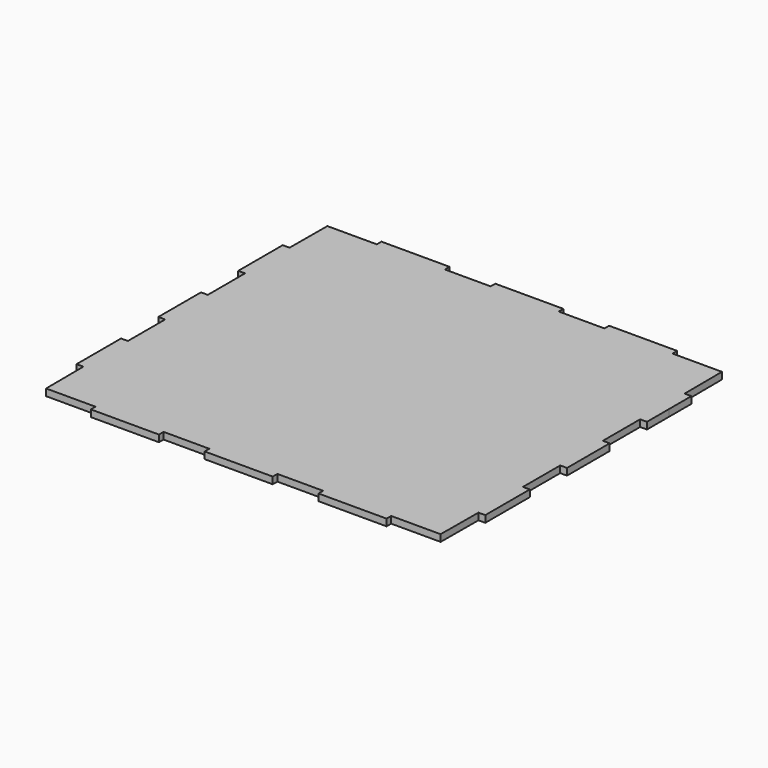
from build123d import *

# Parameters (mm, degrees)
F1_DEPTH = 3


# Not quite as in the source:
# - ends of sketch curves that miss each other by under 0.0002 mm in the source are joined


with BuildPart() as f1:
    # F0 (on Top) → F1 (new body)
    with BuildSketch(Plane.XY):
        Polygon((90.0000515607, 56.7499991818), (87.0000515607, 56.7499991818), (86.8757655059, 77.438837362), (65.1257655059, 77.4387894966), (65.1257655059, 80), (35.1257655059, 80), (35.1257655059, 77.4387894966), (15, 77.4393804423), (15, 80), (-15, 80), (-15, 77.4393804423), (-35.1257655059, 77.4387894966), (-35.1257655059, 80), (-65.1257655059, 80), (-65.1257655059, 77.4387894966), (-86.8757655059, 77.438837362), (-87.0000515607, 56.7499991818), (-90.0000515607, 56.7499991818), (-90.0000505592, 44.4999991818), (-90.0000495577, 32.2499991818), (-87.0000498081, 32.2499991818), (-87.0000523425, 11.7500014042), (-90.0000520921, 11.7500014042), (-90.0000520921, -11.7500014042), (-87.0000523425, -11.7500014042), (-87.0000498081, -32.2499991818), (-90.0000495577, -32.2499991818), (-90.0000515607, -56.7499991818), (-87.0000515607, -56.7499991818), (-86.8757655059, -77.438837362), (-65.1257655059, -77.4387894966), (-65.1257655059, -80), (-35.1257655059, -80), (-35.1257655059, -77.4387894966), (-15, -77.4393804423), (-15, -80), (15, -80), (15, -77.4393804423), (35.1257655059, -77.4387894966), (35.1257655059, -80), (65.1257655059, -80), (65.1257655059, -77.4387894966), (86.8757655059, -77.438837362), (87.0000515607, -56.7499991818), (90.0000515607, -56.7499991818), (90.0000496925, -32.2499991818), (87.0000495577, -32.2499991818), (87.0000524286, -11.7500014042), (90.0000520921, -11.7500014042), (90.0000520921, 11.7500014042), (87.0000523425, 11.7500014042), (87.0000498943, 32.2499991818), (90.0000495577, 32.2499991818), (90.000050694, 44.4999991818), align=None)
    extrude(amount=F1_DEPTH)


solid = f1.part
